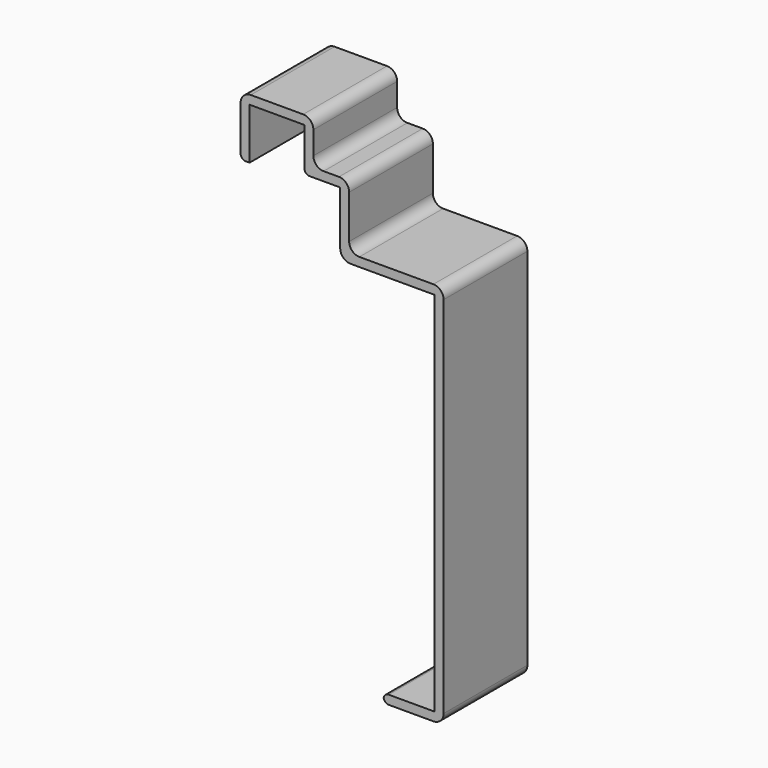
from build123d import *

# Parameters (mm, degrees)
F1_DEPTH    = 41
F2_R        = 4
F3_T1_DEPTH = 51


# Not quite as in the source:
# - a fillet or chamfer that OpenCascade refuses, or shapes differently, is made with other operations: its cross-section is extruded or revolved along the edge and cut away or added


with BuildPart() as f1:
    # F0 (on Front) → F1 (new body)
    with BuildSketch(Plane.XZ):
        Polygon((-42.5, 18.5), (-39, 18.5), (-39, 38.5), (-17.5, 38.5), (-17.5, 21.5), (-3.5, 21.5), (-3.5, -3.5), (0, -3.5), (0, 0), (0, 25), (-14, 25), (-14, 42), (-42.5, 42), align=None)
        Polygon((0, 0), (0, -3.5), (33.5, -3.5), (33.5, -147.2), (13.5, -147.2), (13.5, -150.7), (37, -150.7), (37, 0), align=None)
    extrude(amount=F1_DEPTH)

    # F2
    f2_edges = [f1.edges().sort_by_distance(p)[0] for p in [
        (-42.5, -20.5, 42),
        (-14, -20.5, 42),
        (0, -20.5, 25),
        (0, -20.5, 0),
        (-14, -20.5, 25),
        (37, -20.5, 0),
        (37, -20.5, -150.7),
        (-3.5, -20.5, -3.5),
    ]]
    fillet(f2_edges, radius=F2_R)

    # F3: fillet of radius 2 on 4 edges, made by hand

    # F3_s2 → F3_t1 (cut)
    with BuildSketch(Plane.XZ.offset(-5)):
        with BuildLine():
            ThreePointArc((-40.5, 18.5), (-41.9142135624, 19.0857864376), (-42.5, 20.5))
            Line((-42.5, 20.5), (-42.5, 18.5))
            Line((-42.5, 18.5), (-40.5, 18.5))
        make_face()
        with BuildLine():
            ThreePointArc((15.5, -147.2), (14.0857864376, -147.7857864376), (13.5, -149.2))
            Line((13.5, -149.2), (13.5, -147.2))
            Line((13.5, -147.2), (15.5, -147.2))
        make_face()
        with BuildLine():
            ThreePointArc((13.5, -148.7), (14.0857864376, -150.1142135624), (15.5, -150.7))
            Line((15.5, -150.7), (13.5, -150.7))
            Line((13.5, -150.7), (13.5, -148.7))
        make_face()
        with BuildLine():
            ThreePointArc((-15.5, 21.5), (-16.9142135624, 22.0857864376), (-17.5, 23.5))
            Line((-17.5, 23.5), (-17.5, 21.5))
            Line((-17.5, 21.5), (-15.5, 21.5))
        make_face()
    extrude(amount=F3_T1_DEPTH, mode=Mode.SUBTRACT)


solid = f1.part
